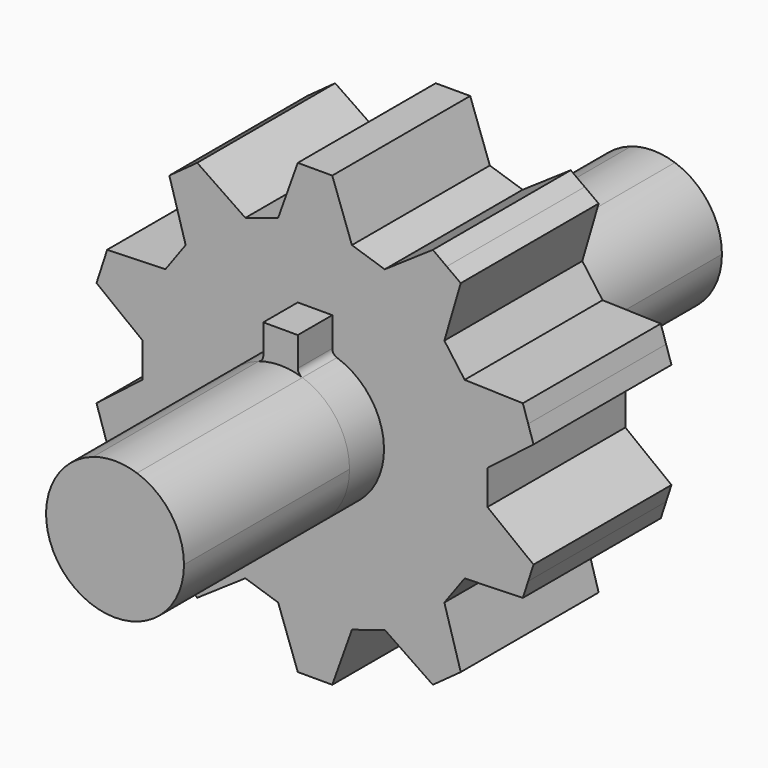
from build123d import *
from build123d import SkipClean  # not in build123d's __all__

# Parameters (mm, degrees)
F1_DEPTH = 25
F3_DEPTH = 25
F4_DEPTH = 37.5
F6_DEPTH = 60


with BuildPart() as f1:
    # F0 (on Front) → F1 (new body, symmetric)
    with BuildSketch(Plane.XZ):
        Polygon((5, 65), (0, 65), (-5, 65), (-10.6955671373, 49.0979107866), (-20.2061323002, 46.0077408429), (-34.1609564271, 55.5250308958), (-38.206041399, 52.5861046344), (-42.2511263709, 49.6471783729), (-37.5119234573, 33.4343475865), (-43.3897759802, 25.3441776427), (-60.2735885873, 24.8413872158), (-61.8186735592, 20.0861046344), (-63.3637585311, 15.3308220529), (-50, 5), (-50, -5), (-63.3637585311, -15.3308220529), (-61.8186735592, -20.0861046344), (-60.2735885873, -24.8413872158), (-43.3897759802, -25.3441776427), (-37.5119234573, -33.4343475865), (-42.2511263709, -49.6471783729), (-38.206041399, -52.5861046344), (-34.1609564271, -55.5250308958), (-20.2061323002, -46.0077408429), (-10.6955671373, -49.0979107866), (-5, -65), (0, -65), (5, -65), (10.6955671373, -49.0979107866), (20.2061323002, -46.0077408429), (34.1609564271, -55.5250308958), (38.206041399, -52.5861046344), (42.2511263709, -49.6471783729), (37.5119234573, -33.4343475865), (43.3897759802, -25.3441776427), (60.2735885873, -24.8413872158), (61.8186735592, -20.0861046344), (63.3637585311, -15.3308220529), (50, -5), (50, 5), (63.3637585311, 15.3308220529), (61.8186735592, 20.0861046344), (60.2735885873, 24.8413872158), (43.3897759802, 25.3441776427), (37.5119234573, 33.4343475865), (42.2511263709, 49.6471783729), (38.206041399, 52.5861046344), (34.1609564271, 55.5250308958), (20.2061323002, 46.0077408429), (10.6955671373, 49.0979107866), align=None)
    extrude(amount=F1_DEPTH, both=True)

    # F2 (on Front) → F3 (cut, symmetric)
    with BuildSketch(Plane.XZ):
        with BuildLine():
            ThreePointArc((-5, 20.8566536146), (-5.3763117182, 19.6889051984), (-6.3636363636, 18.9605941951))
            ThreePointArc((-6.3636363636, 18.9605941951), (0, -20), (6.3636363636, 18.9605941951))
            ThreePointArc((6.3636363636, 18.9605941951), (5.3763117182, 19.6889051984), (5, 20.8566536146))
            Line((5, 20.8566536146), (5, 29.364916731))
            Line((5, 29.364916731), (-5, 29.364916731))
            Line((-5, 29.364916731), (-5, 20.8566536146))
        make_face()
    extrude(amount=F3_DEPTH, both=True, mode=Mode.SUBTRACT)


with BuildPart() as f4:
    # F2 (on Front) → F4 (new body, symmetric)
    with BuildSketch(Plane.XZ):
        with BuildLine():
            ThreePointArc((-5, 20.8566536146), (-5.3763117182, 19.6889051984), (-6.3636363636, 18.9605941951))
            ThreePointArc((-6.3636363636, 18.9605941951), (0, -20), (6.3636363636, 18.9605941951))
            ThreePointArc((6.3636363636, 18.9605941951), (5.3763117182, 19.6889051984), (5, 20.8566536146))
            Line((5, 20.8566536146), (5, 29.364916731))
            Line((5, 29.364916731), (-5, 29.364916731))
            Line((-5, 29.364916731), (-5, 20.8566536146))
        make_face()
    extrude(amount=F4_DEPTH, both=True)

    # F5 (on face) → F6 (join)
    with BuildSketch(Plane.XZ.offset(37.5)):
        with BuildLine():
            ThreePointArc((-6.3636363636, 18.9605941951), (-11.6774841624, -16.2368828177), (20, 0))
            ThreePointArc((20, 0), (16.2368828177, 11.6774841624), (6.3636363636, 18.9605941951))
            ThreePointArc((6.3636363636, 18.9605941951), (0, 20), (-6.3636363636, 18.9605941951))
        make_face()
    with SkipClean():  # cleaning this boolean's faces spoils the solid; the shape is the same uncleaned
        extrude(amount=F6_DEPTH)

    # F7: F4 across plane


with BuildPart() as f4_1:
    add(f4.part, clean=False)
    with SkipClean():  # cleaning this boolean's faces spoils the solid; the shape is the same uncleaned
        add(f4.part.mirror(Plane.XZ), clean=False)


solid = Compound([f1.part, f4_1.part])
